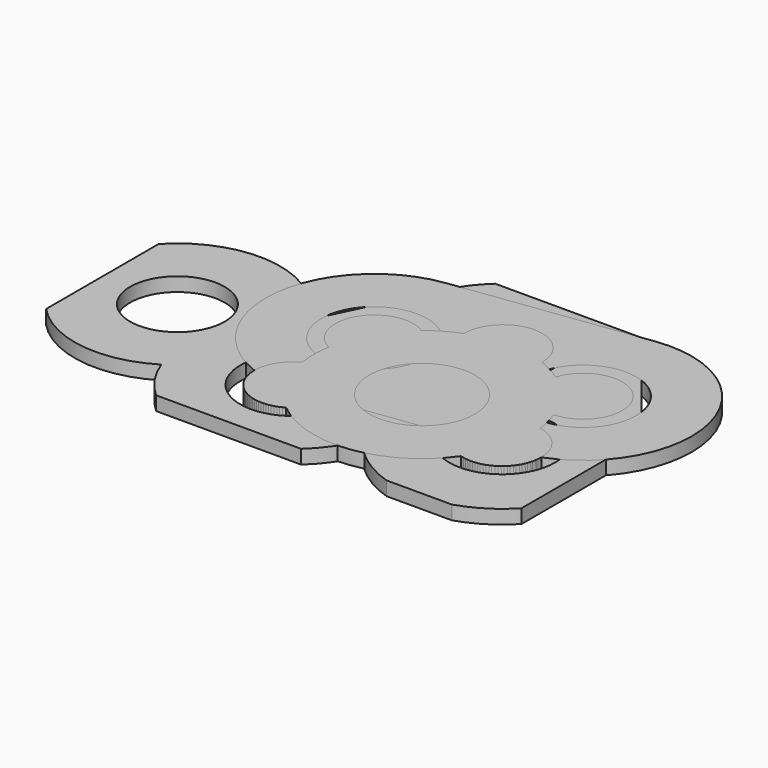
from build123d import *
from build123d import SkipClean  # not in build123d's __all__

# Parameters (mm, degrees)
F1_R      = 17
F1_R_2    = 19
F1_R_3    = 1.5
F2_DEPTH  = 5
F3_R      = 3
F3_R_2    = 1.5
F4_DEPTH  = 3
F5_R      = 19
F6_DEPTH  = 5
F7_R      = 14
F8_DEPTH  = 10
F9_R      = 19
F10_DEPTH = 5
F12_DEPTH = 10


with BuildPart() as f2:
    # F1 (on Top) → F2 (new body)
    with BuildSketch(Plane.XY):
        with BuildLine():
            Line((52.8456293187, 53.3869838042), (34.0990862007, 14.3614873978))
            ThreePointArc((34.0990862007, 14.3614873978), (6.5193782856, 36.4211162208), (-27, 25.2982212813))
            Line((-27, 25.2982212813), (-27, -25.2982212813))
            ThreePointArc((-27, -25.2982212813), (-4.900267379, -36.6740695808), (19.4108786171, -31.4994887468))
            ThreePointArc((19.4108786171, -31.4994887468), (23.7227450142, -39.8901532791), (29.9231903792, -47))
            Line((29.9231903792, -47), (82.0768096208, -47))
            ThreePointArc((82.0768096208, -47), (88.1546210581, -40.0698967965), (92.4362106252, -31.9069247239))
            ThreePointArc((92.4362106252, -31.9069247239), (101.38483284, -41.16001394), (112.8561911904, -47))
            Line((112.8561911904, -47), (136.3244160855, -47))
            ThreePointArc((136.3244160855, -47), (145.3320765814, -42.8394291003), (153, -36.5425053858))
            Line((153, -36.5425053858), (153, 17.2458815256))
            Line((153, 17.2458815256), (118.5725950965, 60.7139717739))
            ThreePointArc((118.5725950965, 60.7139717739), (116.4256095845, 63.2017737192), (114.0768096208, 65.5))
            Line((114.0768096208, 65.5), (61.9231903792, 65.5))
            ThreePointArc((61.9231903792, 65.5), (56.7910966127, 59.8881241095), (52.8456293187, 53.3869838042))
        make_face()
        Circle(F1_R, mode=Mode.SUBTRACT)
        with Locations((56, -18)):
            Circle(F1_R_2, mode=Mode.SUBTRACT)
        with Locations((88, 0)):
            Circle(F1_R_3, mode=Mode.SUBTRACT)
        with Locations((124, -9)):
            Circle(F1_R_2, mode=Mode.SUBTRACT)
        with Locations((56, 18.5)):
            Circle(F1_R_3, mode=Mode.SUBTRACT)
        with Locations((88, 36.5)):
            Circle(F1_R_2, mode=Mode.SUBTRACT)
        with Locations((124, 27.5)):
            Circle(F1_R_3, mode=Mode.SUBTRACT)
    extrude(amount=F2_DEPTH)

    # F3 (on face) → F4 (cut)
    with BuildSketch(Plane.XY.offset(5)):
        with Locations((88, 0)):
            Circle(F3_R)
        with Locations((88, 0)):
            Circle(F3_R_2, mode=Mode.SUBTRACT)
        with Locations((56, 18.5)):
            Circle(F3_R)
        with Locations((56, 18.5)):
            Circle(F3_R_2, mode=Mode.SUBTRACT)
        with Locations((124, 27.5)):
            Circle(F3_R)
        with Locations((124, 27.5)):
            Circle(F3_R_2, mode=Mode.SUBTRACT)
    extrude(amount=-F4_DEPTH, mode=Mode.SUBTRACT)


with BuildPart() as f6:
    # F5 (on Top) → F6 (new body)
    with BuildSketch(Plane.XY):
        with BuildLine():
            Line((118.8828599579, 66.1628358736), (50.8828599579, 57.1628358736))
            ThreePointArc((50.8828599579, 57.1628358736), (17.2702190481, 23.0830194654), (42.0003522717, -17.9006849315))
            ThreePointArc((42.0003522717, -17.9006849315), (55.4541552039, -31.9893550051), (69.9648234925, -18.9918189463))
            Line((69.9648234925, -18.9918189463), (110.7740261985, -13.5906009411))
            ThreePointArc((110.7740261985, -13.5906009411), (126.3766511904, -22.7967941609), (137.9996477283, -8.9006849315))
            ThreePointArc((137.9996477283, -8.9006849315), (161.793620819, 37.1250831366), (118.8828599579, 66.1628358736))
        make_face()
        with Locations((56, 18.5)):
            Circle(F5_R, mode=Mode.SUBTRACT)
        with Locations((124, 27.5)):
            Circle(F5_R, mode=Mode.SUBTRACT)
    extrude(amount=F6_DEPTH)

    # F7 (on face) → F8 (join)
    with BuildSketch(Plane(origin=(0, 0, 0), x_dir=(1, 0, 0), z_dir=(0, 0, -1))):
        with BuildLine():
            ThreePointArc((137.9996477283, 8.9006849315), (137.9999119318, 8.9503421534), (138, 9))
            ThreePointArc((138, 9), (126.3276991621, 22.8051373268), (110.7740261985, 13.5906009411))
            ThreePointArc((110.7740261985, 13.5906009411), (121.6233488096, -4.7967941609), (137.9996477283, 8.9006849315))
        make_face()
        with Locations((88, -36.5)):
            Circle(F7_R)
        with BuildLine():
            ThreePointArc((70, 18), (69.9912031094, 18.4962212735), (69.9648234925, 18.9918189463))
            ThreePointArc((69.9648234925, 18.9918189463), (55.4541552039, 31.9893550051), (42.0003522717, 17.9006849315))
            ThreePointArc((42.0003522717, 17.9006849315), (56.0496578466, 4.0000880682), (70, 18))
        make_face()
    with SkipClean():  # cleaning this boolean's faces spoils the solid; the shape is the same uncleaned
        extrude(amount=F8_DEPTH)


with BuildPart() as f10:
    # F9 (on Top) → F10 (new body)
    with BuildSketch(Plane.XY):
        with BuildLine():
            ThreePointArc((63.4845476575, 30.331379732), (43.8797123644, 25.5070412893), (49.4816005584, 6.1100658307))
            ThreePointArc((49.4816005584, 6.1100658307), (49.0007019381, 0.2339886381), (49.4110577036, -5.6474359174))
            ThreePointArc((49.4110577036, -5.6474359174), (43.7979424803, -24.8636573549), (63.1349363617, -30.0454424209))
            ThreePointArc((63.1349363617, -30.0454424209), (93.2064407376, -38.6509116949), (119.9290177158, -22.3950402479))
            ThreePointArc((119.9290177158, -22.3950402479), (137.581995002, -12.3954987505), (126.71150516, 4.7349095289))
            ThreePointArc((126.71150516, 4.7349095289), (125.9028969833, 9.1853361547), (124.5844277, 13.5122037381))
            ThreePointArc((124.5844277, 13.5122037381), (135.1253941035, 35.9985649402), (110.6583546121, 31.7426994169))
            ThreePointArc((110.6583546121, 31.7426994169), (106.4763765701, 34.3456475967), (101.9996477283, 36.4006849315))
            ThreePointArc((101.9996477283, 36.4006849315), (88, 50.5), (74.0003522717, 36.4006849315))
            ThreePointArc((74.0003522717, 36.4006849315), (68.5048121382, 33.7777685798), (63.4845476575, 30.331379732))
        make_face()
        with Locations((88, 0)):
            Circle(F9_R, mode=Mode.SUBTRACT)
    extrude(amount=F10_DEPTH)

    # F11 (on face) → F12 (join)
    with BuildSketch(Plane(origin=(0, 0, 0), x_dir=(1, 0, 0), z_dir=(0, 0, -1))):
        with BuildLine():
            ThreePointArc((70, -18.5), (63.2367951407, -6.51547681), (49.4816005584, -6.1100658307))
            ThreePointArc((49.4816005584, -6.1100658307), (43.8797123644, -25.5070412893), (63.4845476575, -30.331379732))
            ThreePointArc((63.4845476575, -30.331379732), (68.2634348208, -25.2533818489), (70, -18.5))
        make_face()
        with BuildLine():
            ThreePointArc((49.4110577036, 5.6474359174), (63.2025970264, 5.994892917), (70, 18))
            ThreePointArc((70, 18), (68.1632460524, 24.9322035074), (63.1349363617, 30.0454424209))
            ThreePointArc((63.1349363617, 30.0454424209), (43.7979424803, 24.8636573549), (49.4110577036, 5.6474359174))
        make_face()
        with BuildLine():
            ThreePointArc((101.9996477283, -36.4006849315), (88, -22.5), (74.0003522717, -36.4006849315))
            ThreePointArc((74.0003522717, -36.4006849315), (87.9503421534, -50.4999119318), (102, -36.5))
            ThreePointArc((102, -36.5), (101.9999119318, -36.4503421534), (101.9996477283, -36.4006849315))
        make_face()
        with BuildLine():
            ThreePointArc((138, -27.5), (134.1040088035, -17.8093340735), (124.5844277, -13.5122037381))
            ThreePointArc((124.5844277, -13.5122037381), (112.8746058965, -19.0014350598), (110.6583546121, -31.7426994169))
            ThreePointArc((110.6583546121, -31.7426994169), (126.146737591, -41.3344323236), (138, -27.5))
        make_face()
        with BuildLine():
            ThreePointArc((138, 9), (132.3368533639, 20.2470829991), (119.9290177158, 22.3950402479))
            ThreePointArc((119.9290177158, 22.3950402479), (110.418004998, 5.6045012495), (126.71150516, -4.7349095289))
            ThreePointArc((126.71150516, -4.7349095289), (134.8157540708, 0.1107107213), (138, 9))
        make_face()
    with SkipClean():  # cleaning this boolean's faces spoils the solid; the shape is the same uncleaned
        extrude(amount=F12_DEPTH)


solid = Compound([f2.part, f6.part, f10.part])
